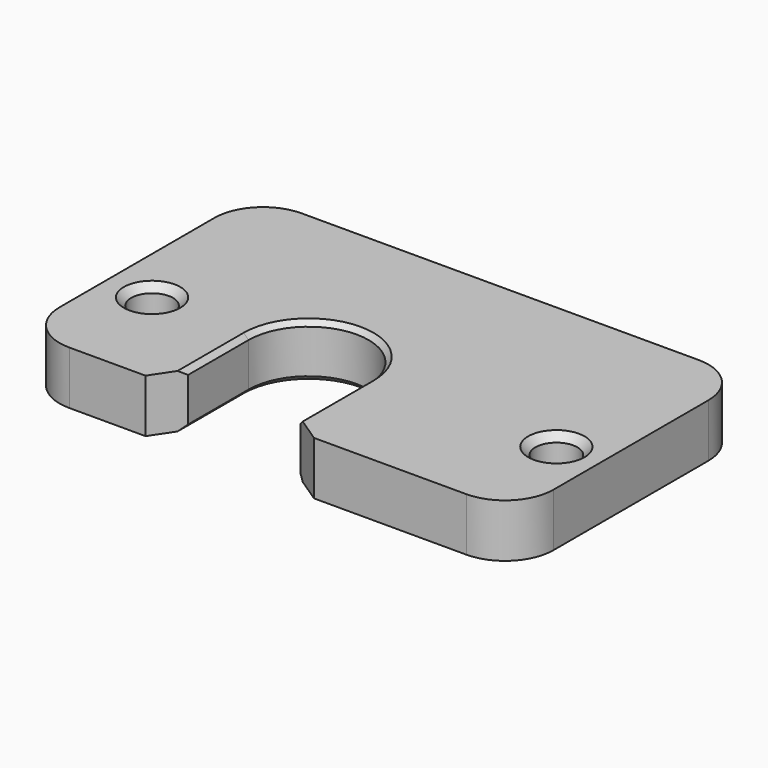
from build123d import *

# Parameters (mm, degrees)
F0_R       = 2.1666665
F1_DEPTH   = 5.5
F2_SIZE    = 0.75
F3_W       = 51
F3_H       = 8
F4_DEPTH   = 5.5
F5_SIZE    = 0.5
F7_R       = 5
F8_SIZE2   = 2
F8_SIZE    = 3
F8_2_SIZE2 = 2
F8_2_SIZE  = 3


with BuildPart() as f1:
    # F0 (on Top) → F1 (new body)
    with BuildSketch(Plane.XY):
        with BuildLine():
            Line((25.5, 11), (-25.5, 11))
            Line((-25.5, 11), (-25.5, -11))
            Line((-25.5, -11), (-10.625, -11))
            Line((-10.625, -11), (-10.625, -0.2))
            ThreePointArc((-10.625, -0.2), (-4.425, 6), (1.775, -0.2))
            Line((1.775, -0.2), (1.775, -11))
            Line((1.775, -11), (25.5, -11))
            Line((25.5, -11), (25.5, 11))
        make_face()
        with Locations((-20.75, 0)):
            Circle(F0_R, mode=Mode.SUBTRACT)
        with Locations((21, 0)):
            Circle(F0_R, mode=Mode.SUBTRACT)
    extrude(amount=F1_DEPTH)

    # F2
    f2_edges = [f1.edges().sort_by_distance(p)[0] for p in [
        (-22.916666, 0, 0),
        (18.833334, 0, 0),
        (18.833334, 0, 5.5),
        (-22.916666, 0, 5.5),
    ]]
    chamfer(f2_edges, length=F2_SIZE)

    # F3 (on Top) → F4 (join, through all)
    with BuildSketch(Plane.XY):
        with Locations((0, 15)):
            Rectangle(F3_W, F3_H)
    extrude(amount=F4_DEPTH)

    # F5
    f5_edges = [f1.edges().sort_by_distance(p)[0] for p in [
        (-4.425, 6, 5.5),
        (-4.425, 6, 0),
        (-10.625, -5.6, 5.5),
        (-10.625, -5.6, 0),
        (1.775, -5.6, 0),
        (1.775, -5.6, 5.5),
    ]]
    chamfer(f5_edges, length=F5_SIZE)

    # F7
    f7_edges = [f1.edges().sort_by_distance(p)[0] for p in [
        (25.5, -11, 2.75),
        (-25.5, -11, 2.75),
        (25.5, 19, 2.75),
        (-25.5, 19, 2.75),
    ]]
    fillet(f7_edges, radius=F7_R)

    # F8
    f8_edges = [f1.edges().sort_by_distance(p)[0] for p in [
        (-10.625, -11, 2.75),
    ]]
    f8_side = f1.faces().sort_by_distance((-10.625, -5.6, 2.75))[0]
    chamfer(f8_edges, length=F8_SIZE, length2=F8_SIZE2, reference=f8_side)

    # F8#2
    f8_2_edges = [f1.edges().sort_by_distance(p)[0] for p in [
        (1.775, -11, 2.75),
    ]]
    f8_2_side = f1.faces().sort_by_distance((11.159877, -11, 2.75))[0]
    chamfer(f8_2_edges, length=F8_2_SIZE, length2=F8_2_SIZE2, reference=f8_2_side)


solid = f1.part
